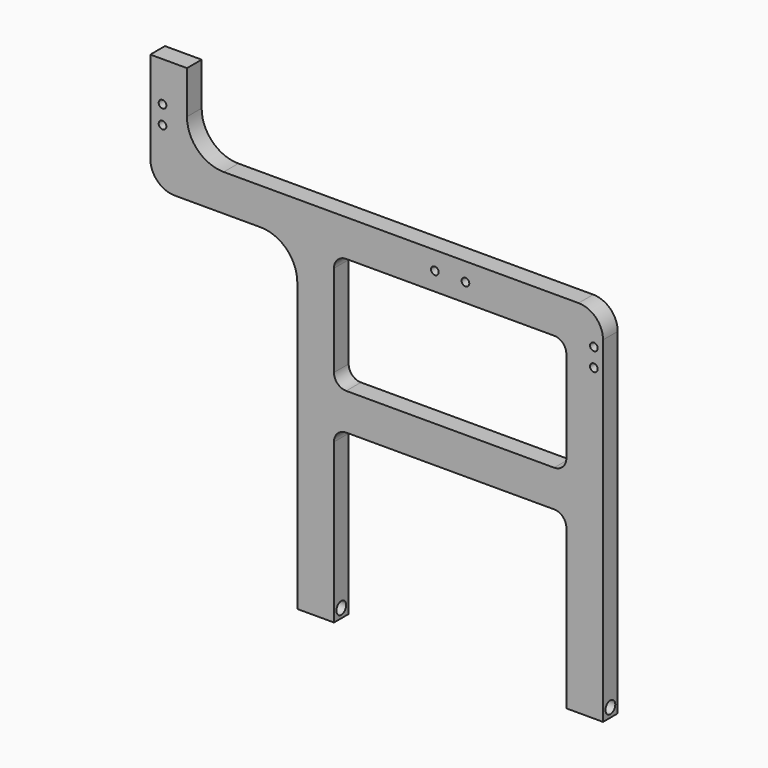
from build123d import *

# Parameters (mm, degrees)
F0_W     = 241.3
F0_H     = 120.65
F1_DEPTH = 9.525
F2_R     = 12.7
F3_R     = 38.1
F5_D     = 12.7
F6_R     = 25.4
F8_D     = 7.9375
F10_D    = 7.9375
F12_D    = 7.9375


# Not quite as in the source:
# - a length typed as a fraction of an inch, garbled in the dataset ("3 / 203.2 mm" for 3/8 in), is restored


with BuildPart() as f1:
    # F0 (on Front) → F1 (new body, symmetric)
    with BuildSketch(Plane.XZ):
        Polygon((-38.1, 0), (0, 0), (0, 374.65), (-432.054, 374.65), (-432.054, 457.2), (-470.154, 457.2), (-470.154, 336.55), (-317.5, 336.55), (-317.5, 0), (-279.4, 0), (-279.4, 177.8), (-38.1, 177.8), align=None)
        with Locations((-158.75, 276.225)):
            Rectangle(F0_W, F0_H, mode=Mode.SUBTRACT)
    extrude(amount=F1_DEPTH, both=True)

    # F2
    f2_edges = [f1.edges().sort_by_distance(p)[0] for p in [
        (-279.4, 0, 336.55),
        (-279.4, 0, 215.9),
        (-38.1, 0, 215.9),
        (-38.1, 0, 336.55),
        (-279.4, 0, 177.8),
        (-38.1, 0, 177.8),
    ]]
    fillet(f2_edges, radius=F2_R)

    # F3
    f3_edges = [f1.edges().sort_by_distance(p)[0] for p in [
        (-317.5, 0, 336.55),
        (-432.054, 0, 374.65),
    ]]
    fillet(f3_edges, radius=F3_R)

    # F5 (through all)
    with Locations(Plane.YZ):
        with Locations((0, 9.525)):
            Hole(F5_D / 2)

    # F6
    f6_edges = [f1.edges().sort_by_distance(p)[0] for p in [
        (-470.154, 0, 336.55),
        (0, 0, 374.65),
    ]]
    fillet(f6_edges, radius=F6_R)

    # F8 (through all)
    with Locations(Plane.XZ.offset(9.525)):
        with Locations((-174.625, 355.6), (-142.875, 355.6)):
            Hole(F8_D / 2)

    # F10 (through all)
    with Locations(Plane(origin=(0, 9.525, 0), x_dir=(-1, 0, 0), z_dir=(0, 1, 0))):
        with Locations((9.525, 320.675), (9.525, 339.725)):
            Hole(F10_D / 2)

    # F12 (through all)
    with Locations(Plane.XZ.offset(9.525)):
        with Locations((-457.454, 415.925), (-457.454, 396.875)):
            Hole(F12_D / 2)


solid = f1.part
